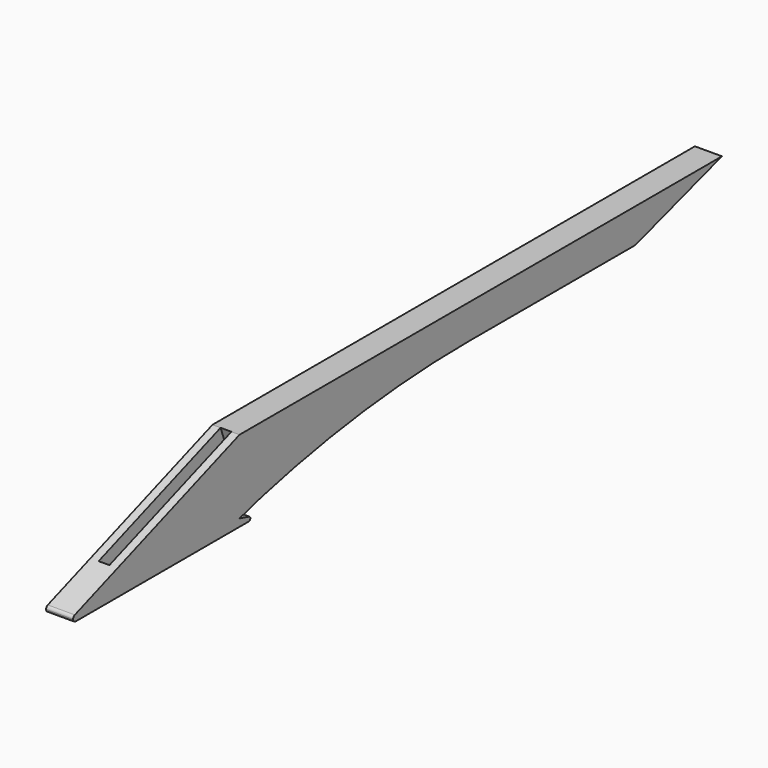
from build123d import *

# Parameters (mm, degrees)
F0_W        = 5
F0_H        = 150
F1_DEPTH    = 15
F2_SIZE2    = 38.4646838724
F2_SIZE     = 14
F3_T1_DEPTH = 7.1006226146
F3_T3_DEPTH = 8
F5_DEPTH    = 25
F6_T1_DEPTH = 6.5227780604
F6_T3_DEPTH = 7
F7_W        = 2
F7_H        = 30
F8_DEPTH    = 3


# Not quite as in the source:
# - a fillet or chamfer that OpenCascade refuses, or shapes differently, is made with other operations: its cross-section is extruded or revolved along the edge and cut away or added


with BuildPart() as f1:
    # F0 (on Top) → F1 (new body)
    with BuildSketch(Plane.XY):
        Rectangle(F0_W, F0_H)
    extrude(amount=F1_DEPTH)

    # F2
    f2_edges = [f1.edges().sort_by_distance(p)[0] for p in [
        (0, -75, 15),
    ]]
    f2_side = f1.faces().sort_by_distance((0, -75, 7.5))[0]
    chamfer(f2_edges, length=F2_SIZE, length2=F2_SIZE2, reference=f2_side)

    # F3: fillet of radius 0.6 on 2 edges, made by hand

    # F3_s2 → F3_t1 (cut)
    with BuildSketch(Plane.YZ.offset(-3.5503113073)):
        with BuildLine():
            ThreePointArc((-75, 0.5798754771), (-74.8914912266, 0.9240213389), (-74.605212086, 1.1436910495))
            Line((-74.605212086, 1.1436910495), (-75, 1))
            Line((-75, 1), (-75, 0.5798754771))
        make_face()
    extrude(amount=F3_T1_DEPTH, mode=Mode.SUBTRACT)

    # F3_s4 → F3_t3 (cut)
    with BuildSketch(Plane.YZ.offset(-4)):
        with BuildLine():
            ThreePointArc((-75, 0.6), (-74.8242640687, 0.1757359313), (-74.4, 0))
            Line((-74.4, 0), (-75, 0))
            Line((-75, 0), (-75, 0.6))
        make_face()
    extrude(amount=F3_T3_DEPTH, mode=Mode.SUBTRACT)

    # F4 (on face) → F5 (cut)
    with BuildSketch(Plane.YZ.offset(2.5)):
        Polygon((55, 8.6759815816), (75, 8.6759815816), (75, 15), align=None)
        with BuildLine():
            ThreePointArc((16.7323419362, 8.6759815816), (46.1873611716, 6.4950955262), (75, 0))
            Line((75, 0), (75, 8.6759815816))
            Line((75, 8.6759815816), (55, 8.6759815816))
            Line((55, 8.6759815816), (16.7323419362, 8.6759815816))
        make_face()
        with BuildLine():
            Line((-31.5353161276, 0), (75, 0))
            ThreePointArc((75, 0), (46.1873611716, 6.4950955262), (16.7323419362, 8.6759815816))
            ThreePointArc((16.7323419362, 8.6759815816), (-7.5818312879, 7.1925324796), (-31.5353161276, 2.7641913859))
            Line((-31.5353161276, 2.7641913859), (-31.5353161276, 2.76))
            Line((-31.5353161276, 2.76), (-31.5353161276, 0))
        make_face()
        Polygon((-34.0353161276, 0.69), (-31.5353161276, 0), (-31.5353161276, 2.76), (-36.5353161276, 1.38), align=None)
        Polygon((-34.0353161276, 0), (-31.5353161276, 0), (-34.0353161276, 0.69), align=None)
    extrude(amount=-F5_DEPTH, mode=Mode.SUBTRACT)

    # F6: fillet of radius 0.4 on 2 edges, made by hand

    # F6_s2 → F6_t1 (cut)
    with BuildSketch(Plane.YZ.offset(-3.2613890302)):
        with BuildLine():
            ThreePointArc((-34.0353161276, 0.3854443879), (-34.1170643339, 0.6277578125), (-34.3288951064, 0.7710277981))
            Line((-34.3288951064, 0.7710277981), (-34.0353161276, 0.69))
            Line((-34.0353161276, 0.69), (-34.0353161276, 0.3854443879))
        make_face()
    extrude(amount=F6_T1_DEPTH, mode=Mode.SUBTRACT)

    # F6_s4 → F6_t3 (cut)
    with BuildSketch(Plane.YZ.offset(-3.5)):
        with BuildLine():
            ThreePointArc((-34.4353161276, 0), (-34.1524734152, 0.1171572875), (-34.0353161276, 0.4))
            Line((-34.0353161276, 0.4), (-34.0353161276, 0))
            Line((-34.0353161276, 0), (-34.4353161276, 0))
        make_face()
    extrude(amount=F6_T3_DEPTH, mode=Mode.SUBTRACT)

    # F7 (on face) → F8 (cut)
    with BuildSketch(Plane(origin=(0, -9.0947271879, 24.9875575848), x_dir=(1, 0, 0), z_dir=(0, -0.3420201433, 0.9396926208))):
        with Locations((0, -44.2016648133)):
            Rectangle(F7_W, F7_H)
    extrude(amount=-F8_DEPTH, mode=Mode.SUBTRACT)


solid = f1.part
